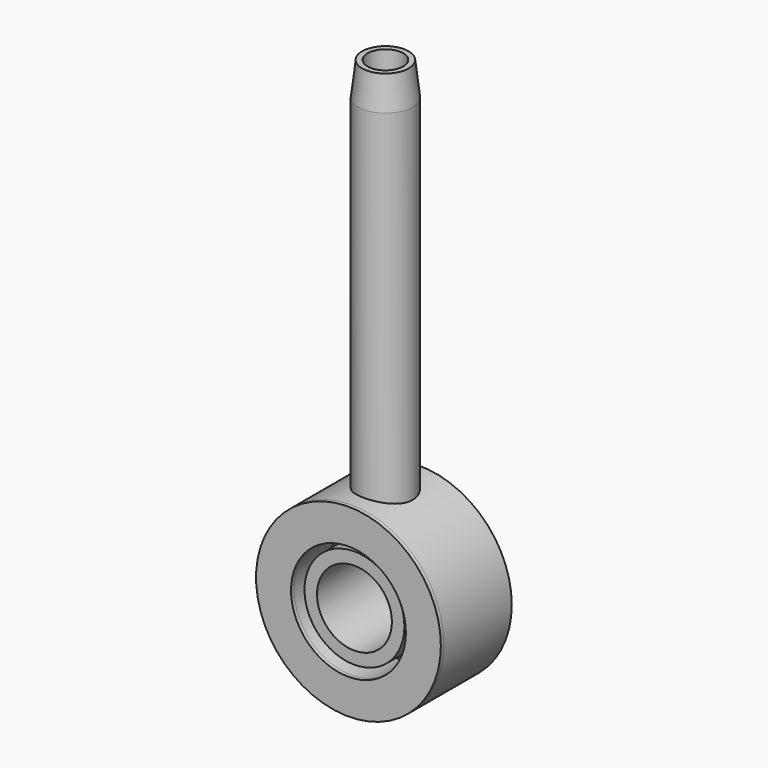
from build123d import *

# Parameters (mm, degrees)
F0_R          = 37
F0_R_2        = 15
F1_DEPTH      = 34
F2_R          = 23
F2_R_2        = 15
F3_DEPTH      = 1.5
F4_R          = 23
F4_R_2        = 20
F5_DEPTH      = 17
F8_END_RADIUS = 20
F7_R          = 7.15
F8_REACH      = 94.2242539419
F9_R          = 10.85
F10_DEPTH     = 10
F11_R         = 10.85
F11_R_2       = 7.15
F12_DEPTH     = 160
F13_SIZE2     = 13.16
F13_SIZE      = 1.5345
F14_R         = 37
F14_R_2       = 23
F15_DEPTH     = 1.5


with BuildPart() as f1:
    # F0 (on Front) → F1 (new body)
    with BuildSketch(Plane.XZ):
        Circle(F0_R)
        Circle(F0_R_2, mode=Mode.SUBTRACT)
    extrude(amount=-F1_DEPTH)

    # F2 (on face) → F3 (cut)
    with BuildSketch(Plane.XZ):
        Circle(F2_R)
        Circle(F2_R_2, mode=Mode.SUBTRACT)
    extrude(amount=-F3_DEPTH, mode=Mode.SUBTRACT)

    # F4 (on face) → F5 (cut)
    with BuildSketch(Plane.XZ):
        Circle(F4_R)
        Circle(F4_R_2, mode=Mode.SUBTRACT)
    extrude(amount=-F5_DEPTH, mode=Mode.SUBTRACT)

    f8_end = (Plane(origin=(0, 9.25, 0), x_dir=(0, 0, -1), z_dir=(0, -1, 0)) * Cylinder(F8_END_RADIUS, 408.5212231395, mode=Mode.PRIVATE)).faces().sort_by_distance((-20, 9.25, 0))[0]
    # F7 (on offset) → F8 (cut, up to the whole of a round face its end follows)
    with BuildSketch(Plane.XY.offset(37)):
        with Locations((0, 17)):
            Circle(F7_R)
    f8_long = extrude(amount=-F8_REACH, mode=Mode.PRIVATE)
    add(split(f8_long, bisect_by=f8_end, keep=Keep.ALL, mode=Mode.PRIVATE).solids().sort_by_distance((0, 17, 37))[0], mode=Mode.SUBTRACT)

    # F9 (on offset) → F10 (cut)
    with BuildSketch(Plane.XY.offset(37)):
        with Locations((0, 17)):
            Circle(F9_R)
    extrude(amount=-F10_DEPTH, mode=Mode.SUBTRACT)


with BuildPart() as f12:
    # F11 (on face) → F12 (new body)
    with BuildSketch(Plane.XY.offset(27)):
        with Locations((0, 17)):
            Circle(F11_R)
        with Locations((0, 17)):
            Circle(F11_R_2, mode=Mode.SUBTRACT)
    extrude(amount=F12_DEPTH)

    # F13
    f13_edges = [f12.edges().sort_by_distance(p)[0] for p in [
        (-10.85, 17, 187),
    ]]
    f13_side = f12.faces().sort_by_distance((-10.543116, 17, 187))[0]
    chamfer(f13_edges, length=F13_SIZE, length2=F13_SIZE2, reference=f13_side)


with BuildPart() as f15:
    # F14 (on face) → F15 (new body)
    with BuildSketch(Plane.XZ):
        Circle(F14_R)
        Circle(F14_R_2, mode=Mode.SUBTRACT)
    extrude(amount=F15_DEPTH)


solid = Compound([f1.part, f12.part, f15.part])
